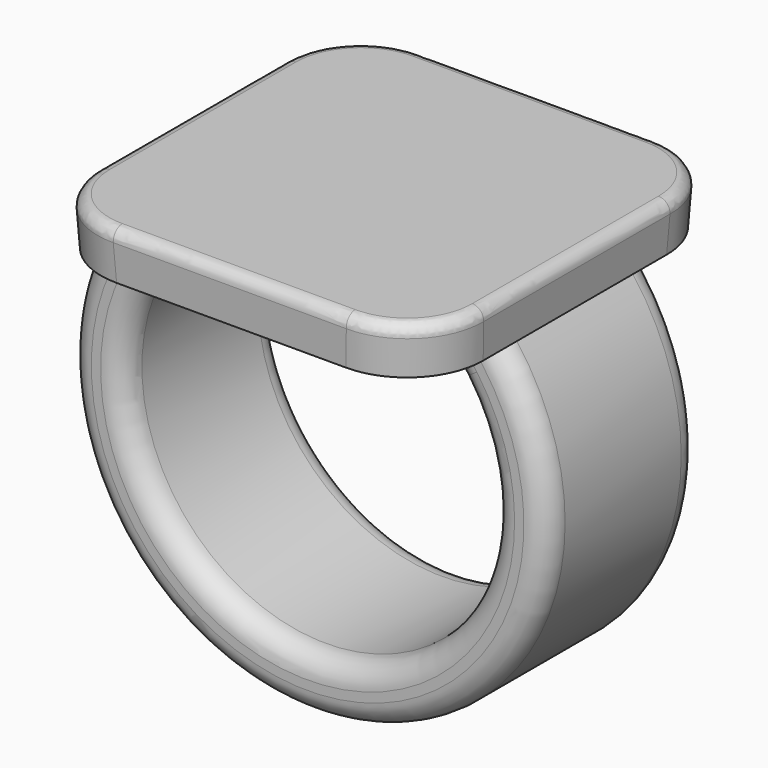
from build123d import *

# Parameters (mm, degrees)
F0_W          = 25.4
F0_H          = 25.4
F1_DEPTH      = 3.175
F1_TAPER      = -3
F3_W          = 5.08
F3_H          = 12.7
F6_DEPTH      = 6.35
F6_DEPTH_BACK = 6.35
F7_R          = 5.08
F8_R          = 1.524
F9_R          = 0.762


with BuildPart() as f1:
    # F0 (on Top) → F1 (new body)
    with BuildSketch(Plane.XY):
        Rectangle(F0_W, F0_H)
    extrude(amount=F1_DEPTH, taper=F1_TAPER)

    # F4: sweep along a path in F2
    with BuildLine(Plane.XZ) as f4_path:
        ThreePointArc((-10.16, 0), (0, -23.5582897328), (10.16, 0))
    # F3 (on face) → F4 (sweep)
    with BuildSketch(Plane(origin=(0, 0, 0), x_dir=(1, 0, 0), z_dir=(0, 0, -1))):
        with Locations((-10.16, 0)):
            Rectangle(F3_W, F3_H)
    sweep(path=f4_path.line)

    # F5 (on Front) → F6 (join, two sides)
    with BuildSketch(Plane.XZ) as f6_sk:
        with BuildLine():
            Line((10.0130578512, -2.535746045), (10.16, 0))
            Line((10.16, 0), (7.62, 0))
            ThreePointArc((7.62, 0), (8.9072265211, -1.1822790439), (10.0130578512, -2.535746045))
        make_face()
    extrude(amount=F6_DEPTH)
    extrude(f6_sk.sketch, amount=-F6_DEPTH_BACK)

    # F7
    f7_edges = [f1.edges().sort_by_distance(p)[0] for p in [
        (12.783197, -12.783197, 1.5875),
        (12.783197, 12.783197, 1.5875),
        (-12.783197, 12.783197, 1.5875),
        (-12.783197, -12.783197, 1.5875),
    ]]
    fillet(f7_edges, radius=F7_R)

    # F8
    f8_edges = [f1.edges().sort_by_distance(p)[0] for p in [
        (-1.743325, 6.35, -21.711017),
        (-1.743325, -6.35, -21.711017),
        (8.907227, -6.35, -1.182279),
        (0, -6.35, -25.501344),
        (8.907227, 6.35, -1.182279),
        (0, 6.35, -25.501344),
    ]]
    fillet(f8_edges, radius=F8_R)

    # F9
    f9_edges = [f1.edges().sort_by_distance(p)[0] for p in [
        (0, -12.866395, 3.175),
        (-11.381378, -11.381378, 3.175),
        (11.381378, -11.381378, 3.175),
        (-12.866395, 0, 3.175),
        (12.866395, 0, 3.175),
        (-11.381378, 11.381378, 3.175),
        (11.381378, 11.381378, 3.175),
        (0, 12.866395, 3.175),
    ]]
    fillet(f9_edges, radius=F9_R)


solid = f1.part
